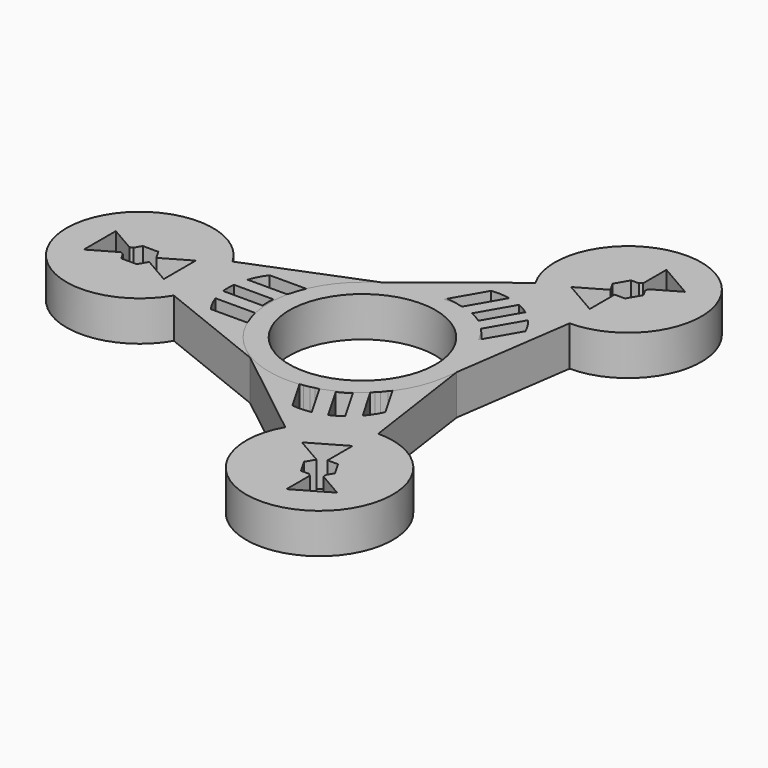
from build123d import *

# Parameters (mm, degrees)
F0_R     = 11
F1_DEPTH = 6
F3_DEPTH = 25
F4_W     = 7.0920773337
F4_H     = 2
F4_W_2   = 8.264102973
F5_DEPTH = 6
F6_COUNT = 3


# Not quite as in the source:
# - a feature names something its author has since deleted; it is built from what else it names


with BuildPart() as f1:
    # F0 (on Top) → F1 (new body)
    with BuildSketch(Plane.XY):
        with BuildLine():
            ThreePointArc((-5.199469469, -12.9986736724), (7.8488033303, -11.5929412266), (14, 0))
            ThreePointArc((14, 0), (7.8488033303, 11.5929412266), (-5.199469469, 12.9986736724))
            ThreePointArc((-5.199469469, 12.9986736724), (-14, 0), (-5.199469469, -12.9986736724))
        make_face()
        Circle(F0_R, mode=Mode.SUBTRACT)
        with BuildLine():
            ThreePointArc((-5.199469469, -12.9986736724), (-14, 0), (-5.199469469, 12.9986736724))
            Line((-5.199469469, 12.9986736724), (-23.9102346195, 5.5143676122))
            ThreePointArc((-23.9102346195, 5.5143676122), (-22.8051712697, 2.8550246743), (-22.4282044575, 0))
            ThreePointArc((-22.4282044575, 0), (-22.8051712697, -2.8550246743), (-23.9102346195, -5.5143676122))
            Line((-23.9102346195, -5.5143676122), (-5.199469469, -12.9986736724))
        make_face()
        with BuildLine():
            ThreePointArc((-22.4282044575, 0), (-22.8051712697, 2.8550246743), (-23.9102346195, 5.5143676122))
            Line((-23.9102346195, 5.5143676122), (-32.6537411335, 2.0169650066))
            Line((-32.6537411335, 2.0169650066), (-32.263709168, 2.0169650066))
            Line((-32.263709168, 2.0169650066), (-31.480499629, 0.6604062919))
            Line((-31.480499629, 0.6604062919), (-27.4282044575, 3))
            Line((-27.4282044575, 3), (-27.4282044575, -3))
            Line((-27.4282044575, -3), (-31.480499629, -0.6604062919))
            Line((-31.480499629, -0.6604062919), (-32.263709168, -2.0169650066))
            Line((-32.263709168, -2.0169650066), (-32.6537411335, -2.0169650066))
            Line((-32.6537411335, -2.0169650066), (-23.9102346195, -5.5143676122))
            ThreePointArc((-23.9102346195, -5.5143676122), (-22.8051712697, -2.8550246743), (-22.4282044575, 0))
        make_face()
        with BuildLine():
            Line((-32.6537411335, 2.0169650066), (-23.9102346195, 5.5143676122))
            ThreePointArc((-23.9102346195, 5.5143676122), (-44.4282044575, 0), (-23.9102346195, -5.5143676122))
            Line((-23.9102346195, -5.5143676122), (-32.6537411335, -2.0169650066))
            Line((-32.6537411335, -2.0169650066), (-34.592699747, -2.0169650066))
            Line((-34.592699747, -2.0169650066), (-35.1749473917, -1.0084825033))
            Line((-35.1749473917, -1.0084825033), (-35.6498043901, -0.818539704))
            Line((-35.6498043901, -0.818539704), (-39.4282044575, -3))
            Line((-39.4282044575, -3), (-39.4282044575, 3))
            Line((-39.4282044575, 3), (-35.6498043901, 0.818539704))
            Line((-35.6498043901, 0.818539704), (-35.1749473917, 1.0084825033))
            Line((-35.1749473917, 1.0084825033), (-34.592699747, 2.0169650066))
            Line((-34.592699747, 2.0169650066), (-32.6537411335, 2.0169650066))
        make_face()
    extrude(amount=F1_DEPTH)

    # F2 (on face) → F3 (cut)
    with BuildSketch(Plane.XY.offset(6)):
        with BuildLine():
            Line((-13.8431219384, 5.5143676122), (-18.3552335948, 5.5143676122))
            ThreePointArc((-18.3552335948, 5.5143676122), (-20.1598162621, 0), (-18.3552335948, -5.5143676122))
            Line((-18.3552335948, -5.5143676122), (-13.8431219384, -5.5143676122))
            Line((-13.8431219384, -5.5143676122), (-12.4311670661, -5.5143676122))
            ThreePointArc((-12.4311670661, -5.5143676122), (-14.2357497334, 0), (-12.4311670661, 5.5143676122))
            Line((-12.4311670661, 5.5143676122), (-13.8431219384, 5.5143676122))
        make_face()
    extrude(amount=-F3_DEPTH, mode=Mode.SUBTRACT)

    # F4 (on face) → F5 (join)
    with BuildSketch(Plane.XY.offset(6)):
        with Locations((-16.8620445766, -2.0143676122)):
            Rectangle(F4_W, F4_H)
        with Locations((-16.0938180052, 2.0143676122)):
            Rectangle(F4_W_2, F4_H)
    extrude(amount=-F5_DEPTH)


with BuildPart() as f6_1:
    # F6: instance of F1
    add(f1.part.rotate(Axis((0, 0, 6), (0, 0, 1)), 1 * 360 / F6_COUNT))


with BuildPart() as f6_2:
    # F6: instance of F1
    add(f1.part.rotate(Axis((0, 0, 6), (0, 0, 1)), 2 * 360 / F6_COUNT))


solid = Compound([f1.part, f6_1.part, f6_2.part])
